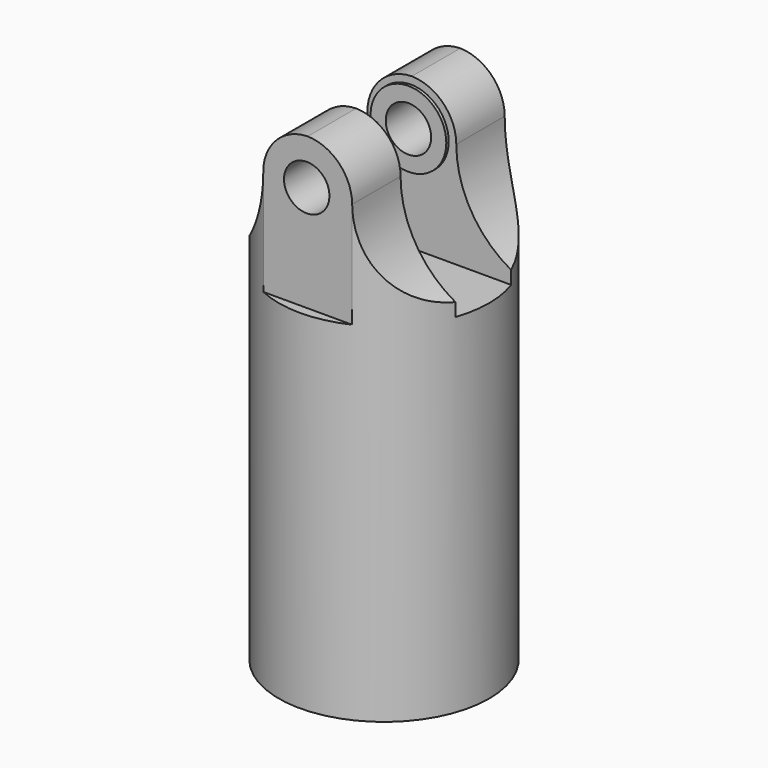
from build123d import *

# Parameters (mm, degrees)
F0_R         = 6.95
F1_DEPTH     = 23
F2_W         = 2.9347061182
F2_H         = 4
F3_DEPTH     = 10
F4_T1_DEPTH  = 19
F4_T3_DEPTH  = 19
F5_T4_DEPTH  = 4
F5_S5_R      = 6.95
F5_T6_DEPTH  = 7
F5_T10_DEPTH = 4
F5_S11_R     = 6.95
F5_T12_DEPTH = 7
F5_T16_DEPTH = 4
F5_S17_R     = 6.95
F5_T18_DEPTH = 7
F5_T22_DEPTH = 4
F5_S23_R     = 6.95
F5_T24_DEPTH = 7
F6_R         = 4.25
F7_DEPTH     = 15
F8_R         = 4
F10_R        = 2.5
F11_DEPTH    = 0.2
F12_R        = 2.5
F13_DEPTH    = 0.2
F9_R         = 1.5
F14_DEPTH    = 13.2510001


# Not quite as in the source:
# - a fillet or chamfer that OpenCascade refuses, or shapes differently, is made with other operations: its cross-section is extruded or revolved along the edge and cut away or added


with BuildPart() as f1:
    # F0 (on Top) → F1 (new body)
    with BuildSketch(Plane.XY):
        with Locations((-16.023524542, 6.9519880981)):
            Circle(F0_R)
    extrude(amount=F1_DEPTH)

    # F2 (on face) → F3 (join)
    with BuildSketch(Plane.XY.offset(23)):
        with Locations((-17.490877601, 11.2519880981)):
            Rectangle(F2_W, F2_H)
        with Locations((-14.5561714829, 11.2519880981)):
            Rectangle(F2_W, F2_H)
        with Locations((-17.490877601, 2.6519880981)):
            Rectangle(F2_W, F2_H)
        with Locations((-14.5561714829, 2.6519880981)):
            Rectangle(F2_W, F2_H)
    extrude(amount=F3_DEPTH)

    # F4: fillet of radius 3 on 4 edges, made by hand

    # F4_s2 → F4_t1 (cut)
    with BuildSketch(Plane.XZ.offset(-12.1519880981)):
        with BuildLine():
            ThreePointArc((-13.0888184238, 30), (-13.9674980802, 32.1213203436), (-16.0888184238, 33))
            Line((-16.0888184238, 33), (-13.0888184238, 33))
            Line((-13.0888184238, 33), (-13.0888184238, 30))
        make_face()
        with BuildLine():
            ThreePointArc((-18.9582306601, 30), (-18.0795510037, 32.1213203436), (-15.9582306601, 33))
            Line((-15.9582306601, 33), (-18.9582306601, 33))
            Line((-18.9582306601, 33), (-18.9582306601, 30))
        make_face()
    extrude(amount=F4_T1_DEPTH, mode=Mode.SUBTRACT)

    # F4_s4 → F4_t3 (cut)
    with BuildSketch(Plane.XZ.offset(-20.7519880981)):
        with BuildLine():
            ThreePointArc((-13.0888184238, 30), (-13.9674980802, 32.1213203436), (-16.0888184238, 33))
            Line((-16.0888184238, 33), (-13.0888184238, 33))
            Line((-13.0888184238, 33), (-13.0888184238, 30))
        make_face()
        with BuildLine():
            ThreePointArc((-18.9582306601, 30), (-18.0795510037, 32.1213203436), (-15.9582306601, 33))
            Line((-15.9582306601, 33), (-18.9582306601, 33))
            Line((-18.9582306601, 33), (-18.9582306601, 30))
        make_face()
    extrude(amount=F4_T3_DEPTH, mode=Mode.SUBTRACT)

    # F5: fillet of radius 7 on 4 edges, made by hand


with BuildPart() as f5_tool2:
    # F5_s3 → F5_t4 (new body)
    with BuildSketch(Plane.XZ.offset(-0.6519880981)):
        with BuildLine():
            ThreePointArc((-13.0888184238, 30), (-11.0385658921, 25.0502525317), (-6.0888184238, 23))
            Line((-6.0888184238, 23), (-6.0888184238, 22.86))
            Line((-6.0888184238, 22.86), (-13.2288184238, 22.86))
            Line((-13.2288184238, 22.86), (-13.2288184238, 30))
            Line((-13.2288184238, 30), (-13.0888184238, 30))
        make_face()
    extrude(amount=-F5_T4_DEPTH)

    # F5_s5 → F5_t6 (intersect, symmetric)
    with BuildSketch(Plane.XY.offset(26.4)):
        with Locations((-16.023524542, 6.9519880981)):
            Circle(F5_S5_R)
    extrude(amount=F5_T6_DEPTH, both=True, mode=Mode.INTERSECT)


with BuildPart() as f1_1:
    add(f1.part)

    # F5_t1: union F5_tool2
    add(f5_tool2.part)


with BuildPart() as f5_tool8:
    # F5_s9 → F5_t10 (new body)
    with BuildSketch(Plane.XZ.offset(-9.2519880981)):
        with BuildLine():
            ThreePointArc((-13.0888184238, 30), (-11.0385658921, 25.0502525317), (-6.0888184238, 23))
            Line((-6.0888184238, 23), (-6.0888184238, 22.86))
            Line((-6.0888184238, 22.86), (-13.2288184238, 22.86))
            Line((-13.2288184238, 22.86), (-13.2288184238, 30))
            Line((-13.2288184238, 30), (-13.0888184238, 30))
        make_face()
    extrude(amount=-F5_T10_DEPTH)

    # F5_s11 → F5_t12 (intersect, symmetric)
    with BuildSketch(Plane.XY.offset(26.4)):
        with Locations((-16.023524542, 6.9519880981)):
            Circle(F5_S11_R)
    extrude(amount=F5_T12_DEPTH, both=True, mode=Mode.INTERSECT)


with BuildPart() as f1_2:
    add(f1_1.part)

    # F5_t7: union F5_tool8
    add(f5_tool8.part)


with BuildPart() as f5_tool14:
    # F5_s15 → F5_t16 (new body)
    with BuildSketch(Plane.XZ.offset(-13.2519880981)):
        with BuildLine():
            ThreePointArc((-18.9582306601, 30), (-21.0084831918, 25.0502525317), (-25.9582306601, 23))
            Line((-25.9582306601, 23), (-25.9582306601, 22.86))
            Line((-25.9582306601, 22.86), (-18.8182306601, 22.86))
            Line((-18.8182306601, 22.86), (-18.8182306601, 30))
            Line((-18.8182306601, 30), (-18.9582306601, 30))
        make_face()
    extrude(amount=F5_T16_DEPTH)

    # F5_s17 → F5_t18 (intersect, symmetric)
    with BuildSketch(Plane.XY.offset(26.4)):
        with Locations((-16.023524542, 6.9519880981)):
            Circle(F5_S17_R)
    extrude(amount=F5_T18_DEPTH, both=True, mode=Mode.INTERSECT)


with BuildPart() as f1_3:
    add(f1_2.part)

    # F5_t13: union F5_tool14
    add(f5_tool14.part)


with BuildPart() as f5_tool20:
    # F5_s21 → F5_t22 (new body)
    with BuildSketch(Plane.XZ.offset(-4.6519880981)):
        with BuildLine():
            ThreePointArc((-18.9582306601, 30), (-21.0084831918, 25.0502525317), (-25.9582306601, 23))
            Line((-25.9582306601, 23), (-25.9582306601, 22.86))
            Line((-25.9582306601, 22.86), (-18.8182306601, 22.86))
            Line((-18.8182306601, 22.86), (-18.8182306601, 30))
            Line((-18.8182306601, 30), (-18.9582306601, 30))
        make_face()
    extrude(amount=F5_T22_DEPTH)

    # F5_s23 → F5_t24 (intersect, symmetric)
    with BuildSketch(Plane.XY.offset(26.4)):
        with Locations((-16.023524542, 6.9519880981)):
            Circle(F5_S23_R)
    extrude(amount=F5_T24_DEPTH, both=True, mode=Mode.INTERSECT)


with BuildPart() as f1_4:
    add(f1_3.part)

    # F5_t19: union F5_tool20
    add(f5_tool20.part)

    # F6 (on face) → F7 (cut)
    with BuildSketch(Plane(origin=(0, 0, 0), x_dir=(1, 0, 0), z_dir=(0, 0, -1))):
        with Locations((-16.023524542, -6.9519880981)):
            Circle(F6_R)
    extrude(amount=-F7_DEPTH, mode=Mode.SUBTRACT)

    # F8
    f8_edges = [f1_4.edges().sort_by_distance(p)[0] for p in [
        (-20.273525, 6.951988, 15),
    ]]
    fillet(f8_edges, radius=F8_R)

    # F10 (on face) → F11 (join)
    with BuildSketch(Plane(origin=(0, 4.6519880981, 0), x_dir=(-1, 0, 0), z_dir=(0, 1, 0))):
        with Locations((15.9582306601, 30)):
            Circle(F10_R)
    extrude(amount=F11_DEPTH)

    # F12 (on face) → F13 (join)
    with BuildSketch(Plane.XZ.offset(-9.2519880981)):
        with Locations((-16.0888184238, 30)):
            Circle(F12_R)
    extrude(amount=F13_DEPTH)

    # F9 (on face) → F14 (cut, through all)
    with BuildSketch(Plane(origin=(0, 13.2519880981, 0), x_dir=(-1, 0, 0), z_dir=(0, 1, 0))):
        with Locations((16.0888184238, 30)):
            Circle(F9_R)
    extrude(amount=-F14_DEPTH, mode=Mode.SUBTRACT)


solid = f1_4.part
